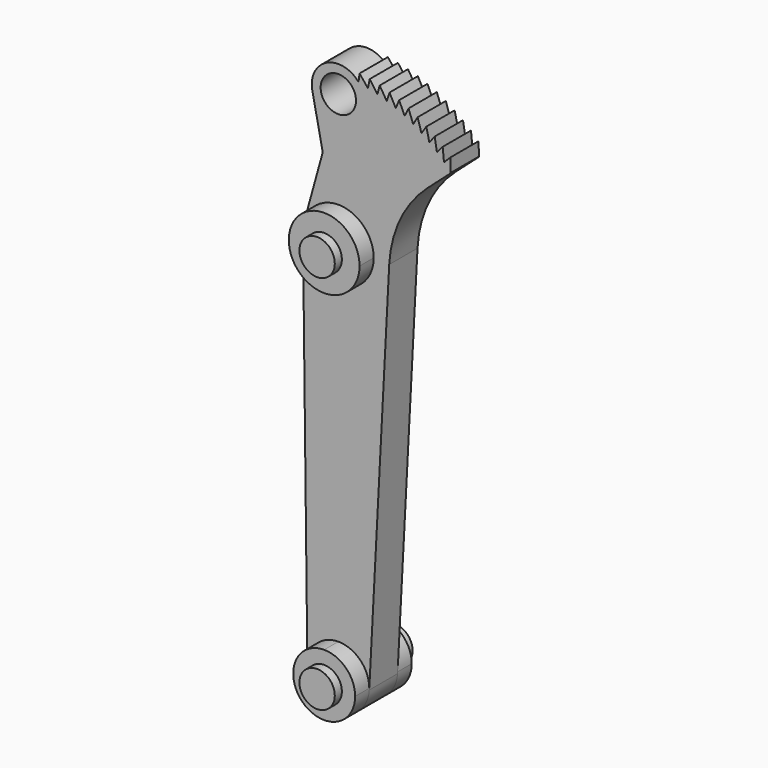
from build123d import *

# Parameters (mm, degrees)
F0_R     = 1.5875
F1_DEPTH = 3.175
F5_DEPTH = 1.5875
F6_R     = 1.5875
F7_DEPTH = 0.79375
F8_R     = 1.5875
F9_DEPTH = 1.5875
F10_R    = 10.31875


# Not quite as in the source:
# - a feature of the source that left no trace in its solid (it failed there, or was rolled back) is left out
# - a pattern or mirror of a feature is missing from the dataset's text; its kind, count and spacing are read off the source's solid


with BuildPart() as f1:
    # F0 (on Front) → F1 (new body)
    with BuildSketch(Plane.XZ):
        with BuildLine():
            Line((-3.1747853497, 34.0943313953), (-2.777937181, -0.0323037791))
            ThreePointArc((-2.777937181, -0.0323037791), (-0.0565749778, -2.7775488812), (2.7743176762, -0.1453958284))
            Line((2.7743176762, -0.1453958284), (4.7932141006, 38.3774428034))
            Line((4.7932141006, 38.3774428034), (10.1004515544, 43.0789965018))
            ThreePointArc((10.1004515544, 43.0789965018), (10.0925772968, 43.0878759884), (10.0846956661, 43.0967489312))
            Line((10.0846956661, 43.0967489312), (10.0430595374, 44.2934156835))
            Line((10.0430595374, 44.2934156835), (9.4851117853, 43.7288509233))
            Line((9.4851117853, 43.7288509233), (9.3663379592, 44.9203356649))
            Line((9.3663379592, 44.9203356649), (8.8459858503, 44.3209420168))
            Line((8.8459858503, 44.3209420168), (8.6505703336, 45.5022785002))
            Line((8.6505703336, 45.5022785002), (8.1699830928, 44.8705546947))
            Line((8.1699830928, 44.8705546947), (7.8987405265, 46.0368182075))
            Line((7.8987405265, 46.0368182075), (7.4599216084, 45.3753977516))
            Line((7.4599216084, 45.3753977516), (7.1139827386, 46.5217264172))
            Line((7.1139827386, 46.5217264172), (6.7187614754, 45.8333666162))
            Line((6.7187614754, 45.8333666162), (6.2995684394, 46.9549816615))
            Line((6.2995684394, 46.9549816615), (5.949592415, 46.2425521248))
            Line((5.949592415, 46.2425521248), (5.4588927295, 47.334777802))
            Line((5.4588927295, 47.334777802), (5.1556209112, 46.6012484796))
            Line((5.1556209112, 46.6012484796), (4.5954601871, 47.6595315582))
            Line((4.5954601871, 47.6595315582), (4.3401568434, 46.9079603605))
            Line((4.3401568434, 46.9079603605), (3.7128702582, 47.9278891087))
            Line((3.7128702582, 47.9278891087), (3.5065996883, 47.1614091582))
            Line((3.5065996883, 47.1614091582), (2.8148022515, 48.1387317342))
            Line((2.8148022515, 48.1387317342), (2.6584243486, 47.3605383046))
            Line((2.6584243486, 47.3605383046), (1.905, 48.2911804818))
            Line((1.905, 48.2911804818), (1.8099761367, 47.5848648397))
            ThreePointArc((1.8099761367, 47.5848648397), (-1.0450737271, 48.1771664384), (-2.33313898, 45.56125))
            Line((-2.33313898, 45.56125), (-1.3985654512, 40.9827934547))
            Line((-1.3985654512, 40.9827934547), (-3.0600295024, 34.9779166667))
            ThreePointArc((-3.0600295024, 34.9779166667), (-3.1485567794, 34.5401695607), (-3.1747853497, 34.0943313953))
        make_face()
        with Locations((0, 46.0375)):
            Circle(F0_R, mode=Mode.SUBTRACT)
    extrude(amount=F1_DEPTH)

    # F4 (on face) → F5 (join)
    with BuildSketch(Plane.XZ.offset(3.175)):
        with BuildLine():
            ThreePointArc((0, 2.778125), (-1.9644310265, -1.9644310265), (2.778125, 0))
            ThreePointArc((2.778125, 0), (1.9644310265, 1.9644310265), (0, 2.778125))
        make_face()
        with BuildLine():
            ThreePointArc((3.175, 34.13125), (-2.2450640303, 36.3763140303), (0, 30.95625))
            ThreePointArc((0, 30.95625), (2.2450640303, 31.8861859697), (3.175, 34.13125))
        make_face()
    f5 = extrude(amount=F5_DEPTH)

    # F5_copies: F5 across plane
    add(f5.mirror(Plane.ZX.offset(-1.5875)))

    # F6 (on face) → F7 (join)
    with BuildSketch(Plane.XZ.offset(4.7625)):
        Circle(F6_R)
        with Locations((0, 34.13125)):
            Circle(F6_R)
    extrude(amount=F7_DEPTH)

    # F8 (on face) → F9 (join)
    with BuildSketch(Plane(origin=(0, 1.5875, 0), x_dir=(-1, 0, 0), z_dir=(0, 1, 0))):
        Circle(F8_R)
        with Locations((0, 34.13125)):
            Circle(F8_R)
    extrude(amount=F9_DEPTH)

    # F10
    f10_edges = [f1.edges().sort_by_distance(p)[0] for p in [
        (4.793214, -1.5875, 38.377443),
    ]]
    fillet(f10_edges, radius=F10_R)


solid = f1.part
